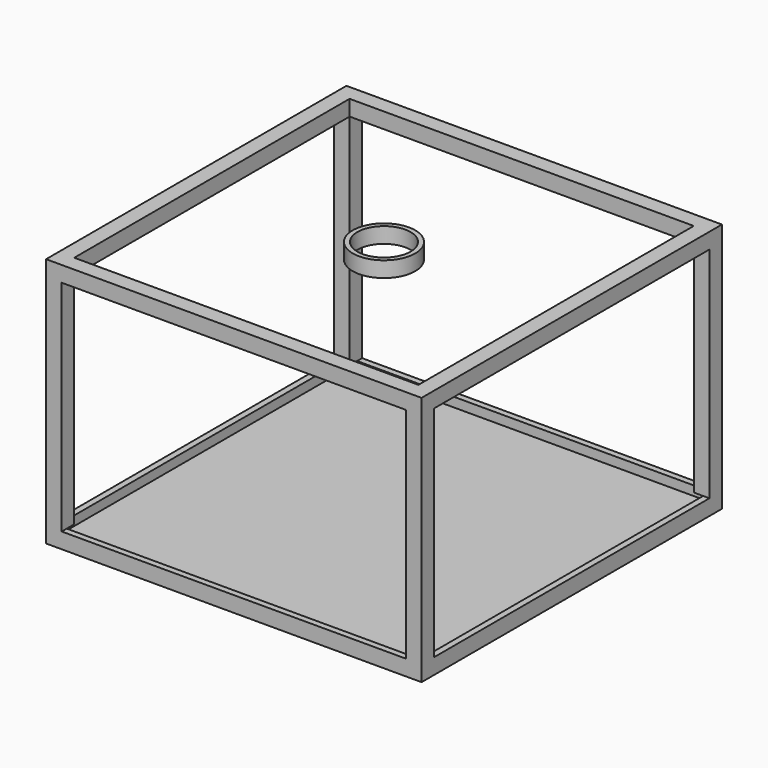
from build123d import *

# Parameters (mm, degrees)
F0_W      = 152.4
F0_H      = 152.4
F1_DEPTH  = 6.35
F2_W      = 6.35
F2_H      = 6.35
F3_DEPTH  = 95.25
F4_W      = 6.35
F4_H      = 6.35
F5_DEPTH  = 95.25
F6_W      = 6.35
F6_H      = 6.35
F7_DEPTH  = 95.25
F8_W      = 6.35
F8_H      = 6.35
F9_DEPTH  = 95.25
F10_W     = 6.35
F10_H     = 6.35
F11_DEPTH = 139.7
F12_W     = 6.35
F12_H     = 6.35
F13_DEPTH = 139.7
F14_W     = 6.35
F14_H     = 6.35
F15_DEPTH = 139.7
F16_W     = 6.35
F16_H     = 6.35
F17_DEPTH = 139.7
F18_T     = -2.54
F22_R     = 12.7
F23_DEPTH = 6.35
F24_R     = 10.795
F25_DEPTH = 25.4


# Not quite as in the source:
# - a shell that OpenCascade refuses in one call is made with other operations: the cavity is built on its own and cut out
# - the program builds the solid bodies; features that only make, move or delete a surface that nothing else refers to are left out


with BuildPart() as f1:
    # F0 (on Top) → F1 (new body)
    with BuildSketch(Plane.XY):
        Rectangle(F0_W, F0_H)
    extrude(amount=F1_DEPTH)

    # F2 (on face) → F3 (join)
    with BuildSketch(Plane.XY.offset(6.35)):
        with Locations((73.025, -73.025)):
            Rectangle(F2_W, F2_H)
    extrude(amount=F3_DEPTH)

    # F4 (on face) → F5 (join)
    with BuildSketch(Plane.XY.offset(6.35)):
        with Locations((73.025, 73.025)):
            Rectangle(F4_W, F4_H)
    extrude(amount=F5_DEPTH)

    # F6 (on face) → F7 (join)
    with BuildSketch(Plane.XY.offset(6.35)):
        with Locations((-73.025, 73.025)):
            Rectangle(F6_W, F6_H)
    extrude(amount=F7_DEPTH)

    # F8 (on face) → F9 (join)
    with BuildSketch(Plane.XY.offset(6.35)):
        with Locations((-73.025, -73.025)):
            Rectangle(F8_W, F8_H)
    extrude(amount=F9_DEPTH)

    # F10 (on face) → F11 (join)
    with BuildSketch(Plane(origin=(69.85, 0, 0), x_dir=(0, -1, 0), z_dir=(-1, 0, 0))):
        with Locations((-73.025, 98.425)):
            Rectangle(F10_W, F10_H)
    extrude(amount=F11_DEPTH)

    # F12 (on face) → F13 (join)
    with BuildSketch(Plane.XZ.offset(-69.85)):
        with Locations((-73.025, 98.425)):
            Rectangle(F12_W, F12_H)
    extrude(amount=F13_DEPTH)

    # F14 (on face) → F15 (join)
    with BuildSketch(Plane.YZ.offset(-69.85)):
        with Locations((-73.025, 98.425)):
            Rectangle(F14_W, F14_H)
    extrude(amount=F15_DEPTH)

    # F16 (on face) → F17 (join)
    with BuildSketch(Plane.XZ.offset(-69.85)):
        with Locations((73.025, 98.425)):
            Rectangle(F16_W, F16_H)
    extrude(amount=F17_DEPTH)

    # F18: a shell. OpenCascade refuses it in one call, so the cavity is built on its own and cut out:
    # the body offset inwards by the wall thickness, plus a prism from it out through each open face.
    f18_core = offset(f1.part, amount=F18_T, kind=Kind.INTERSECTION, mode=Mode.PRIVATE)
    f18_exits = [f18_core.faces().sort_by_distance(p)[0] for p in [
        (0, 0, 3.81),
    ]]
    add(f18_core, mode=Mode.SUBTRACT)
    extrude(f18_exits, amount=-F18_T, mode=Mode.SUBTRACT)


with BuildPart() as f23:
    # F22 (on offset) → F23 (new body)
    with BuildSketch(Plane.XY.offset(95.25)):
        Circle(F22_R)
    extrude(amount=F23_DEPTH)

    # F24 (on face) → F25 (cut)
    with BuildSketch(Plane.XY.offset(101.6)):
        Circle(F24_R)
    extrude(amount=-F25_DEPTH, mode=Mode.SUBTRACT)


solid = Compound([f1.part, f23.part])
